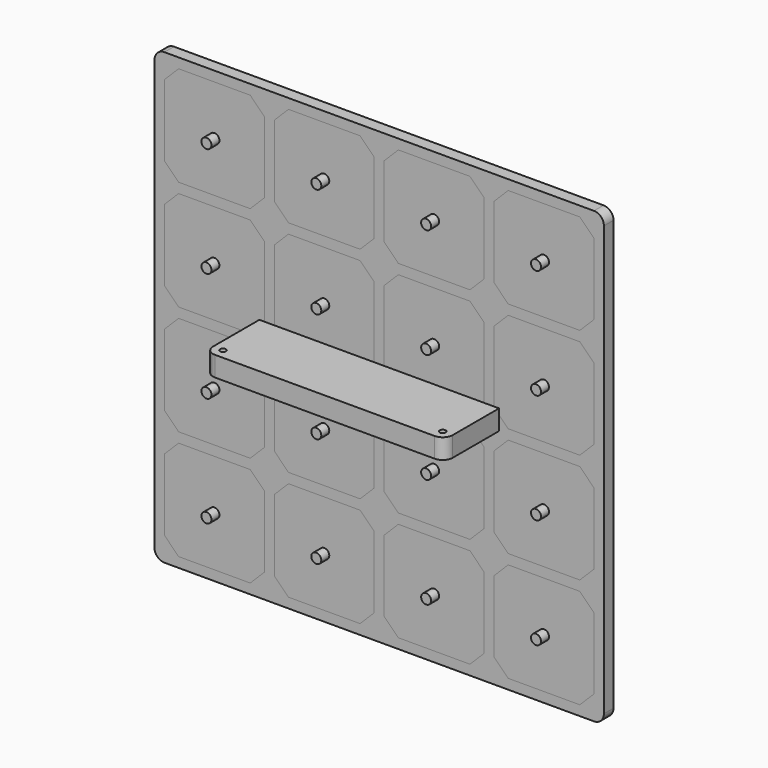
from build123d import *

# Parameters (mm, degrees)
F0_R          = 2.5
F1_DEPTH      = 6
F0_W          = 225
F0_H          = 225
F2_DEPTH      = 6
F3_R          = 5
F4_D          = 5
F4_2_D        = 5
F4_3_D        = 5
F4_4_D        = 5
F4_5_D        = 5
F4_6_D        = 5
F4_7_D        = 5
F4_8_D        = 5
F4_9_D        = 5
F4_10_D       = 5
F4_11_D       = 5
F4_12_D       = 5
F4_13_D       = 5
F4_14_D       = 5
F4_15_D       = 5
F5_R          = 2.5
F6_DEPTH      = 25
F6_DEPTH_BACK = 5
F8_DEPTH      = 10
F9_D          = 3
F10_T         = -3


with BuildPart() as f1:
    # F0 (on Front) → F1 (new body)
    with BuildSketch(Plane.XZ):
        Polygon((-107.5, 100.4289321881), (-107.5, 82.5), (-107.5, 64.5710678119), (-100.4289321881, 57.5), (-82.5, 57.5), (-64.5710678119, 57.5), (-57.5, 64.5710678119), (-57.5, 82.5), (-57.5, 100.4289321881), (-64.5710678119, 107.5), (-82.5, 107.5), (-100.4289321881, 107.5), align=None)
        with Locations((-82.5, 82.5)):
            Circle(F0_R, mode=Mode.SUBTRACT)
    extrude(amount=F1_DEPTH)


with BuildPart() as f1b:
    # F0 (on Front) → F1, piece 2 (new body)
    with BuildSketch(Plane.XZ):
        Polygon((-45.4289321881, 107.5), (-52.5, 100.4289321881), (-52.5, 82.5), (-52.5, 64.5710678119), (-45.4289321881, 57.5), (-27.5, 57.5), (-9.5710678119, 57.5), (-2.5, 64.5710678119), (-2.5, 82.5), (-2.5, 100.4289321881), (-9.5710678119, 107.5), (-27.5, 107.5), align=None)
    extrude(amount=F1_DEPTH)

    # F4 (through all)
    with Locations(Plane(origin=(0, 0, 0), x_dir=(1, 0, 0), z_dir=(0, 1, 0))):
        with Locations((-82.5, -82.5), (-27.5, -82.5), (27.5, -82.5), (82.5, -82.5), (-82.5, -27.5), (-27.5, -27.5), (27.5, -27.5), (82.5, -27.5), (-82.5, 27.5), (-27.5, 27.5), (27.5, 27.5), (82.5, 27.5), (-82.5, 82.5), (-27.5, 82.5), (27.5, 82.5), (82.5, 82.5)):
            Hole(F4_D / 2)


with BuildPart() as f1c:
    # F0 (on Front) → F1, piece 3 (new body)
    with BuildSketch(Plane.XZ):
        Polygon((9.5710678119, 107.5), (2.5, 100.4289321881), (2.5, 82.5), (2.5, 64.5710678119), (9.5710678119, 57.5), (27.5, 57.5), (45.4289321881, 57.5), (52.5, 64.5710678119), (52.5, 82.5), (52.5, 100.4289321881), (45.4289321881, 107.5), (27.5, 107.5), align=None)
    extrude(amount=F1_DEPTH)

    # F4#2 (through all)
    with Locations(Plane(origin=(0, 0, 0), x_dir=(1, 0, 0), z_dir=(0, 1, 0))):
        with Locations((-82.5, -82.5), (-27.5, -82.5), (27.5, -82.5), (82.5, -82.5), (-82.5, -27.5), (-27.5, -27.5), (27.5, -27.5), (82.5, -27.5), (-82.5, 27.5), (-27.5, 27.5), (27.5, 27.5), (82.5, 27.5), (-82.5, 82.5), (-27.5, 82.5), (27.5, 82.5), (82.5, 82.5)):
            Hole(F4_2_D / 2)


with BuildPart() as f1d:
    # F0 (on Front) → F1, piece 4 (new body)
    with BuildSketch(Plane.XZ):
        Polygon((64.5710678119, 107.5), (57.5, 100.4289321881), (57.5, 82.5), (57.5, 64.5710678119), (64.5710678119, 57.5), (82.5, 57.5), (100.4289321881, 57.5), (107.5, 64.5710678119), (107.5, 82.5), (107.5, 100.4289321881), (100.4289321881, 107.5), (82.5, 107.5), align=None)
    extrude(amount=F1_DEPTH)

    # F4#3 (through all)
    with Locations(Plane(origin=(0, 0, 0), x_dir=(1, 0, 0), z_dir=(0, 1, 0))):
        with Locations((-82.5, -82.5), (-27.5, -82.5), (27.5, -82.5), (82.5, -82.5), (-82.5, -27.5), (-27.5, -27.5), (27.5, -27.5), (82.5, -27.5), (-82.5, 27.5), (-27.5, 27.5), (27.5, 27.5), (82.5, 27.5), (-82.5, 82.5), (-27.5, 82.5), (27.5, 82.5), (82.5, 82.5)):
            Hole(F4_3_D / 2)


with BuildPart() as f1e:
    # F0 (on Front) → F1, piece 5 (new body)
    with BuildSketch(Plane.XZ):
        Polygon((64.5710678119, 52.5), (57.5, 45.4289321881), (57.5, 27.5), (57.5, 9.5710678119), (64.5710678119, 2.5), (82.5, 2.5), (100.4289321881, 2.5), (107.5, 9.5710678119), (107.5, 27.5), (107.5, 45.4289321881), (100.4289321881, 52.5), (82.5, 52.5), align=None)
    extrude(amount=F1_DEPTH)

    # F4#4 (through all)
    with Locations(Plane(origin=(0, 0, 0), x_dir=(1, 0, 0), z_dir=(0, 1, 0))):
        with Locations((-82.5, -82.5), (-27.5, -82.5), (27.5, -82.5), (82.5, -82.5), (-82.5, -27.5), (-27.5, -27.5), (27.5, -27.5), (82.5, -27.5), (-82.5, 27.5), (-27.5, 27.5), (27.5, 27.5), (82.5, 27.5), (-82.5, 82.5), (-27.5, 82.5), (27.5, 82.5), (82.5, 82.5)):
            Hole(F4_4_D / 2)


with BuildPart() as f1f:
    # F0 (on Front) → F1, piece 6 (new body)
    with BuildSketch(Plane.XZ):
        Polygon((9.5710678119, 52.5), (2.5, 45.4289321881), (2.5, 27.5), (2.5, 9.5710678119), (9.5710678119, 2.5), (27.5, 2.5), (45.4289321881, 2.5), (52.5, 9.5710678119), (52.5, 27.5), (52.5, 45.4289321881), (45.4289321881, 52.5), (27.5, 52.5), align=None)
    extrude(amount=F1_DEPTH)

    # F4#5 (through all)
    with Locations(Plane(origin=(0, 0, 0), x_dir=(1, 0, 0), z_dir=(0, 1, 0))):
        with Locations((-82.5, -82.5), (-27.5, -82.5), (27.5, -82.5), (82.5, -82.5), (-82.5, -27.5), (-27.5, -27.5), (27.5, -27.5), (82.5, -27.5), (-82.5, 27.5), (-27.5, 27.5), (27.5, 27.5), (82.5, 27.5), (-82.5, 82.5), (-27.5, 82.5), (27.5, 82.5), (82.5, 82.5)):
            Hole(F4_5_D / 2)


with BuildPart() as f1g:
    # F0 (on Front) → F1, piece 7 (new body)
    with BuildSketch(Plane.XZ):
        Polygon((-45.4289321881, 52.5), (-52.5, 45.4289321881), (-52.5, 27.5), (-52.5, 9.5710678119), (-45.4289321881, 2.5), (-27.5, 2.5), (-9.5710678119, 2.5), (-2.5, 9.5710678119), (-2.5, 27.5), (-2.5, 45.4289321881), (-9.5710678119, 52.5), (-27.5, 52.5), align=None)
    extrude(amount=F1_DEPTH)

    # F4#6 (through all)
    with Locations(Plane(origin=(0, 0, 0), x_dir=(1, 0, 0), z_dir=(0, 1, 0))):
        with Locations((-82.5, -82.5), (-27.5, -82.5), (27.5, -82.5), (82.5, -82.5), (-82.5, -27.5), (-27.5, -27.5), (27.5, -27.5), (82.5, -27.5), (-82.5, 27.5), (-27.5, 27.5), (27.5, 27.5), (82.5, 27.5), (-82.5, 82.5), (-27.5, 82.5), (27.5, 82.5), (82.5, 82.5)):
            Hole(F4_6_D / 2)


with BuildPart() as f1h:
    # F0 (on Front) → F1, piece 8 (new body)
    with BuildSketch(Plane.XZ):
        Polygon((-100.4289321881, 52.5), (-107.5, 45.4289321881), (-107.5, 27.5), (-107.5, 9.5710678119), (-100.4289321881, 2.5), (-82.5, 2.5), (-64.5710678119, 2.5), (-57.5, 9.5710678119), (-57.5, 27.5), (-57.5, 45.4289321881), (-64.5710678119, 52.5), (-82.5, 52.5), align=None)
    extrude(amount=F1_DEPTH)

    # F4#7 (through all)
    with Locations(Plane(origin=(0, 0, 0), x_dir=(1, 0, 0), z_dir=(0, 1, 0))):
        with Locations((-82.5, -82.5), (-27.5, -82.5), (27.5, -82.5), (82.5, -82.5), (-82.5, -27.5), (-27.5, -27.5), (27.5, -27.5), (82.5, -27.5), (-82.5, 27.5), (-27.5, 27.5), (27.5, 27.5), (82.5, 27.5), (-82.5, 82.5), (-27.5, 82.5), (27.5, 82.5), (82.5, 82.5)):
            Hole(F4_7_D / 2)


with BuildPart() as f1i:
    # F0 (on Front) → F1, piece 9 (new body)
    with BuildSketch(Plane.XZ):
        Polygon((-100.4289321881, -2.5), (-107.5, -9.5710678119), (-107.5, -27.5), (-107.5, -45.4289321881), (-100.4289321881, -52.5), (-82.5, -52.5), (-64.5710678119, -52.5), (-57.5, -45.4289321881), (-57.5, -27.5), (-57.5, -9.5710678119), (-64.5710678119, -2.5), (-82.5, -2.5), align=None)
    extrude(amount=F1_DEPTH)

    # F4#8 (through all)
    with Locations(Plane(origin=(0, 0, 0), x_dir=(1, 0, 0), z_dir=(0, 1, 0))):
        with Locations((-82.5, -82.5), (-27.5, -82.5), (27.5, -82.5), (82.5, -82.5), (-82.5, -27.5), (-27.5, -27.5), (27.5, -27.5), (82.5, -27.5), (-82.5, 27.5), (-27.5, 27.5), (27.5, 27.5), (82.5, 27.5), (-82.5, 82.5), (-27.5, 82.5), (27.5, 82.5), (82.5, 82.5)):
            Hole(F4_8_D / 2)


with BuildPart() as f1j:
    # F0 (on Front) → F1, piece 10 (new body)
    with BuildSketch(Plane.XZ):
        Polygon((-45.4289321881, -2.5), (-52.5, -9.5710678119), (-52.5, -27.5), (-52.5, -45.4289321881), (-45.4289321881, -52.5), (-27.5, -52.5), (-9.5710678119, -52.5), (-2.5, -45.4289321881), (-2.5, -27.5), (-2.5, -9.5710678119), (-9.5710678119, -2.5), (-27.5, -2.5), align=None)
    extrude(amount=F1_DEPTH)

    # F4#9 (through all)
    with Locations(Plane(origin=(0, 0, 0), x_dir=(1, 0, 0), z_dir=(0, 1, 0))):
        with Locations((-82.5, -82.5), (-27.5, -82.5), (27.5, -82.5), (82.5, -82.5), (-82.5, -27.5), (-27.5, -27.5), (27.5, -27.5), (82.5, -27.5), (-82.5, 27.5), (-27.5, 27.5), (27.5, 27.5), (82.5, 27.5), (-82.5, 82.5), (-27.5, 82.5), (27.5, 82.5), (82.5, 82.5)):
            Hole(F4_9_D / 2)


with BuildPart() as f1k:
    # F0 (on Front) → F1, piece 11 (new body)
    with BuildSketch(Plane.XZ):
        Polygon((9.5710678119, -2.5), (2.5, -9.5710678119), (2.5, -27.5), (2.5, -45.4289321881), (9.5710678119, -52.5), (27.5, -52.5), (45.4289321881, -52.5), (52.5, -45.4289321881), (52.5, -27.5), (52.5, -9.5710678119), (45.4289321881, -2.5), (27.5, -2.5), align=None)
    extrude(amount=F1_DEPTH)

    # F4#10 (through all)
    with Locations(Plane(origin=(0, 0, 0), x_dir=(1, 0, 0), z_dir=(0, 1, 0))):
        with Locations((-82.5, -82.5), (-27.5, -82.5), (27.5, -82.5), (82.5, -82.5), (-82.5, -27.5), (-27.5, -27.5), (27.5, -27.5), (82.5, -27.5), (-82.5, 27.5), (-27.5, 27.5), (27.5, 27.5), (82.5, 27.5), (-82.5, 82.5), (-27.5, 82.5), (27.5, 82.5), (82.5, 82.5)):
            Hole(F4_10_D / 2)


with BuildPart() as f1l:
    # F0 (on Front) → F1, piece 12 (new body)
    with BuildSketch(Plane.XZ):
        Polygon((64.5710678119, -2.5), (57.5, -9.5710678119), (57.5, -27.5), (57.5, -45.4289321881), (64.5710678119, -52.5), (82.5, -52.5), (100.4289321881, -52.5), (107.5, -45.4289321881), (107.5, -27.5), (107.5, -9.5710678119), (100.4289321881, -2.5), (82.5, -2.5), align=None)
    extrude(amount=F1_DEPTH)

    # F4#11 (through all)
    with Locations(Plane(origin=(0, 0, 0), x_dir=(1, 0, 0), z_dir=(0, 1, 0))):
        with Locations((-82.5, -82.5), (-27.5, -82.5), (27.5, -82.5), (82.5, -82.5), (-82.5, -27.5), (-27.5, -27.5), (27.5, -27.5), (82.5, -27.5), (-82.5, 27.5), (-27.5, 27.5), (27.5, 27.5), (82.5, 27.5), (-82.5, 82.5), (-27.5, 82.5), (27.5, 82.5), (82.5, 82.5)):
            Hole(F4_11_D / 2)


with BuildPart() as f1m:
    # F0 (on Front) → F1, piece 13 (new body)
    with BuildSketch(Plane.XZ):
        Polygon((64.5710678119, -57.5), (57.5, -64.5710678119), (57.5, -82.5), (57.5, -100.4289321881), (64.5710678119, -107.5), (82.5, -107.5), (100.4289321881, -107.5), (107.5, -100.4289321881), (107.5, -82.5), (107.5, -64.5710678119), (100.4289321881, -57.5), (82.5, -57.5), align=None)
    extrude(amount=F1_DEPTH)

    # F4#12 (through all)
    with Locations(Plane(origin=(0, 0, 0), x_dir=(1, 0, 0), z_dir=(0, 1, 0))):
        with Locations((-82.5, -82.5), (-27.5, -82.5), (27.5, -82.5), (82.5, -82.5), (-82.5, -27.5), (-27.5, -27.5), (27.5, -27.5), (82.5, -27.5), (-82.5, 27.5), (-27.5, 27.5), (27.5, 27.5), (82.5, 27.5), (-82.5, 82.5), (-27.5, 82.5), (27.5, 82.5), (82.5, 82.5)):
            Hole(F4_12_D / 2)


with BuildPart() as f1n:
    # F0 (on Front) → F1, piece 14 (new body)
    with BuildSketch(Plane.XZ):
        Polygon((9.5710678119, -57.5), (2.5, -64.5710678119), (2.5, -82.5), (2.5, -100.4289321881), (9.5710678119, -107.5), (27.5, -107.5), (45.4289321881, -107.5), (52.5, -100.4289321881), (52.5, -82.5), (52.5, -64.5710678119), (45.4289321881, -57.5), (27.5, -57.5), align=None)
    extrude(amount=F1_DEPTH)

    # F4#13 (through all)
    with Locations(Plane(origin=(0, 0, 0), x_dir=(1, 0, 0), z_dir=(0, 1, 0))):
        with Locations((-82.5, -82.5), (-27.5, -82.5), (27.5, -82.5), (82.5, -82.5), (-82.5, -27.5), (-27.5, -27.5), (27.5, -27.5), (82.5, -27.5), (-82.5, 27.5), (-27.5, 27.5), (27.5, 27.5), (82.5, 27.5), (-82.5, 82.5), (-27.5, 82.5), (27.5, 82.5), (82.5, 82.5)):
            Hole(F4_13_D / 2)


with BuildPart() as f1o:
    # F0 (on Front) → F1, piece 15 (new body)
    with BuildSketch(Plane.XZ):
        Polygon((-45.4289321881, -57.5), (-52.5, -64.5710678119), (-52.5, -82.5), (-52.5, -100.4289321881), (-45.4289321881, -107.5), (-27.5, -107.5), (-9.5710678119, -107.5), (-2.5, -100.4289321881), (-2.5, -82.5), (-2.5, -64.5710678119), (-9.5710678119, -57.5), (-27.5, -57.5), align=None)
    extrude(amount=F1_DEPTH)

    # F4#14 (through all)
    with Locations(Plane(origin=(0, 0, 0), x_dir=(1, 0, 0), z_dir=(0, 1, 0))):
        with Locations((-82.5, -82.5), (-27.5, -82.5), (27.5, -82.5), (82.5, -82.5), (-82.5, -27.5), (-27.5, -27.5), (27.5, -27.5), (82.5, -27.5), (-82.5, 27.5), (-27.5, 27.5), (27.5, 27.5), (82.5, 27.5), (-82.5, 82.5), (-27.5, 82.5), (27.5, 82.5), (82.5, 82.5)):
            Hole(F4_14_D / 2)


with BuildPart() as f1p:
    # F0 (on Front) → F1, piece 16 (new body)
    with BuildSketch(Plane.XZ):
        Polygon((-100.4289321881, -57.5), (-107.5, -64.5710678119), (-107.5, -82.5), (-107.5, -100.4289321881), (-100.4289321881, -107.5), (-82.5, -107.5), (-64.5710678119, -107.5), (-57.5, -100.4289321881), (-57.5, -82.5), (-57.5, -64.5710678119), (-64.5710678119, -57.5), (-82.5, -57.5), align=None)
    extrude(amount=F1_DEPTH)

    # F4#15 (through all)
    with Locations(Plane(origin=(0, 0, 0), x_dir=(1, 0, 0), z_dir=(0, 1, 0))):
        with Locations((-82.5, -82.5), (-27.5, -82.5), (27.5, -82.5), (82.5, -82.5), (-82.5, -27.5), (-27.5, -27.5), (27.5, -27.5), (82.5, -27.5), (-82.5, 27.5), (-27.5, 27.5), (27.5, 27.5), (82.5, 27.5), (-82.5, 82.5), (-27.5, 82.5), (27.5, 82.5), (82.5, 82.5)):
            Hole(F4_15_D / 2)


with BuildPart() as f2:
    # F0 (on Front) → F2 (new body)
    with BuildSketch(Plane.XZ):
        Rectangle(F0_W, F0_H)
        Polygon((-107.5, -82.5), (-107.5, -64.5710678119), (-100.4289321881, -57.5), (-82.5, -57.5), (-64.5710678119, -57.5), (-57.5, -64.5710678119), (-57.5, -82.5), (-57.5, -100.4289321881), (-64.5710678119, -107.5), (-82.5, -107.5), (-100.4289321881, -107.5), (-107.5, -100.4289321881), align=None, mode=Mode.SUBTRACT)
        Polygon((-52.5, -82.5), (-52.5, -64.5710678119), (-45.4289321881, -57.5), (-27.5, -57.5), (-9.5710678119, -57.5), (-2.5, -64.5710678119), (-2.5, -82.5), (-2.5, -100.4289321881), (-9.5710678119, -107.5), (-27.5, -107.5), (-45.4289321881, -107.5), (-52.5, -100.4289321881), align=None, mode=Mode.SUBTRACT)
        Polygon((-107.5, -27.5), (-107.5, -9.5710678119), (-100.4289321881, -2.5), (-82.5, -2.5), (-64.5710678119, -2.5), (-57.5, -9.5710678119), (-57.5, -27.5), (-57.5, -45.4289321881), (-64.5710678119, -52.5), (-82.5, -52.5), (-100.4289321881, -52.5), (-107.5, -45.4289321881), align=None, mode=Mode.SUBTRACT)
        Polygon((-52.5, -27.5), (-52.5, -9.5710678119), (-45.4289321881, -2.5), (-27.5, -2.5), (-9.5710678119, -2.5), (-2.5, -9.5710678119), (-2.5, -27.5), (-2.5, -45.4289321881), (-9.5710678119, -52.5), (-27.5, -52.5), (-45.4289321881, -52.5), (-52.5, -45.4289321881), align=None, mode=Mode.SUBTRACT)
        Polygon((2.5, -82.5), (2.5, -64.5710678119), (9.5710678119, -57.5), (27.5, -57.5), (45.4289321881, -57.5), (52.5, -64.5710678119), (52.5, -82.5), (52.5, -100.4289321881), (45.4289321881, -107.5), (27.5, -107.5), (9.5710678119, -107.5), (2.5, -100.4289321881), align=None, mode=Mode.SUBTRACT)
        Polygon((57.5, -82.5), (57.5, -64.5710678119), (64.5710678119, -57.5), (82.5, -57.5), (100.4289321881, -57.5), (107.5, -64.5710678119), (107.5, -82.5), (107.5, -100.4289321881), (100.4289321881, -107.5), (82.5, -107.5), (64.5710678119, -107.5), (57.5, -100.4289321881), align=None, mode=Mode.SUBTRACT)
        Polygon((2.5, -27.5), (2.5, -9.5710678119), (9.5710678119, -2.5), (27.5, -2.5), (45.4289321881, -2.5), (52.5, -9.5710678119), (52.5, -27.5), (52.5, -45.4289321881), (45.4289321881, -52.5), (27.5, -52.5), (9.5710678119, -52.5), (2.5, -45.4289321881), align=None, mode=Mode.SUBTRACT)
        Polygon((57.5, -27.5), (57.5, -9.5710678119), (64.5710678119, -2.5), (82.5, -2.5), (100.4289321881, -2.5), (107.5, -9.5710678119), (107.5, -27.5), (107.5, -45.4289321881), (100.4289321881, -52.5), (82.5, -52.5), (64.5710678119, -52.5), (57.5, -45.4289321881), align=None, mode=Mode.SUBTRACT)
        Polygon((-107.5, 27.5), (-107.5, 45.4289321881), (-100.4289321881, 52.5), (-82.5, 52.5), (-64.5710678119, 52.5), (-57.5, 45.4289321881), (-57.5, 27.5), (-57.5, 9.5710678119), (-64.5710678119, 2.5), (-82.5, 2.5), (-100.4289321881, 2.5), (-107.5, 9.5710678119), align=None, mode=Mode.SUBTRACT)
        Polygon((-52.5, 27.5), (-52.5, 45.4289321881), (-45.4289321881, 52.5), (-27.5, 52.5), (-9.5710678119, 52.5), (-2.5, 45.4289321881), (-2.5, 27.5), (-2.5, 9.5710678119), (-9.5710678119, 2.5), (-27.5, 2.5), (-45.4289321881, 2.5), (-52.5, 9.5710678119), align=None, mode=Mode.SUBTRACT)
        Polygon((-107.5, 64.5710678119), (-107.5, 82.5), (-107.5, 100.4289321881), (-100.4289321881, 107.5), (-82.5, 107.5), (-64.5710678119, 107.5), (-57.5, 100.4289321881), (-57.5, 82.5), (-57.5, 64.5710678119), (-64.5710678119, 57.5), (-82.5, 57.5), (-100.4289321881, 57.5), align=None, mode=Mode.SUBTRACT)
        Polygon((-52.5, 82.5), (-52.5, 100.4289321881), (-45.4289321881, 107.5), (-27.5, 107.5), (-9.5710678119, 107.5), (-2.5, 100.4289321881), (-2.5, 82.5), (-2.5, 64.5710678119), (-9.5710678119, 57.5), (-27.5, 57.5), (-45.4289321881, 57.5), (-52.5, 64.5710678119), align=None, mode=Mode.SUBTRACT)
        Polygon((2.5, 27.5), (2.5, 45.4289321881), (9.5710678119, 52.5), (27.5, 52.5), (45.4289321881, 52.5), (52.5, 45.4289321881), (52.5, 27.5), (52.5, 9.5710678119), (45.4289321881, 2.5), (27.5, 2.5), (9.5710678119, 2.5), (2.5, 9.5710678119), align=None, mode=Mode.SUBTRACT)
        Polygon((57.5, 27.5), (57.5, 45.4289321881), (64.5710678119, 52.5), (82.5, 52.5), (100.4289321881, 52.5), (107.5, 45.4289321881), (107.5, 27.5), (107.5, 9.5710678119), (100.4289321881, 2.5), (82.5, 2.5), (64.5710678119, 2.5), (57.5, 9.5710678119), align=None, mode=Mode.SUBTRACT)
        Polygon((2.5, 82.5), (2.5, 100.4289321881), (9.5710678119, 107.5), (27.5, 107.5), (45.4289321881, 107.5), (52.5, 100.4289321881), (52.5, 82.5), (52.5, 64.5710678119), (45.4289321881, 57.5), (27.5, 57.5), (9.5710678119, 57.5), (2.5, 64.5710678119), align=None, mode=Mode.SUBTRACT)
        Polygon((57.5, 82.5), (57.5, 100.4289321881), (64.5710678119, 107.5), (82.5, 107.5), (100.4289321881, 107.5), (107.5, 100.4289321881), (107.5, 82.5), (107.5, 64.5710678119), (100.4289321881, 57.5), (82.5, 57.5), (64.5710678119, 57.5), (57.5, 64.5710678119), align=None, mode=Mode.SUBTRACT)
    extrude(amount=F2_DEPTH)

    # F3
    f3_edges = [f2.edges().sort_by_distance(p)[0] for p in [
        (-112.5, -3, 112.5),
        (112.5, -3, 112.5),
        (112.5, -3, -112.5),
        (-112.5, -3, -112.5),
    ]]
    fillet(f3_edges, radius=F3_R)


with BuildPart() as f6:
    # F5 (on face) → F6 (new body, two sides)
    with BuildSketch(Plane.XZ.offset(6)) as f6_sk:
        with Locations((-82.5, 82.5)):
            Circle(F5_R)
    extrude(amount=-F6_DEPTH)
    extrude(f6_sk.sketch, amount=F6_DEPTH_BACK)


with BuildPart() as f6b:
    # F5 (on face) → F6, piece 2 (new body, two sides)
    with BuildSketch(Plane.XZ.offset(6)) as f6_2_sk:
        with Locations((-82.5, 27.5)):
            Circle(F5_R)
    extrude(amount=-F6_DEPTH)
    extrude(f6_2_sk.sketch, amount=F6_DEPTH_BACK)


with BuildPart() as f6c:
    # F5 (on face) → F6, piece 3 (new body, two sides)
    with BuildSketch(Plane.XZ.offset(6)) as f6_3_sk:
        with Locations((-82.5, -27.5)):
            Circle(F5_R)
    extrude(amount=-F6_DEPTH)
    extrude(f6_3_sk.sketch, amount=F6_DEPTH_BACK)


with BuildPart() as f6d:
    # F5 (on face) → F6, piece 4 (new body, two sides)
    with BuildSketch(Plane.XZ.offset(6)) as f6_4_sk:
        with Locations((-82.5, -82.5)):
            Circle(F5_R)
    extrude(amount=-F6_DEPTH)
    extrude(f6_4_sk.sketch, amount=F6_DEPTH_BACK)


with BuildPart() as f6e:
    # F5 (on face) → F6, piece 5 (new body, two sides)
    with BuildSketch(Plane.XZ.offset(6)) as f6_5_sk:
        with Locations((-27.5, 82.5)):
            Circle(F5_R)
    extrude(amount=-F6_DEPTH)
    extrude(f6_5_sk.sketch, amount=F6_DEPTH_BACK)


with BuildPart() as f6f:
    # F5 (on face) → F6, piece 6 (new body, two sides)
    with BuildSketch(Plane.XZ.offset(6)) as f6_6_sk:
        with Locations((-27.5, 27.5)):
            Circle(F5_R)
    extrude(amount=-F6_DEPTH)
    extrude(f6_6_sk.sketch, amount=F6_DEPTH_BACK)


with BuildPart() as f6g:
    # F5 (on face) → F6, piece 7 (new body, two sides)
    with BuildSketch(Plane.XZ.offset(6)) as f6_7_sk:
        with Locations((-27.5, -27.5)):
            Circle(F5_R)
    extrude(amount=-F6_DEPTH)
    extrude(f6_7_sk.sketch, amount=F6_DEPTH_BACK)


with BuildPart() as f6h:
    # F5 (on face) → F6, piece 8 (new body, two sides)
    with BuildSketch(Plane.XZ.offset(6)) as f6_8_sk:
        with Locations((-27.5, -82.5)):
            Circle(F5_R)
    extrude(amount=-F6_DEPTH)
    extrude(f6_8_sk.sketch, amount=F6_DEPTH_BACK)


with BuildPart() as f6i:
    # F5 (on face) → F6, piece 9 (new body, two sides)
    with BuildSketch(Plane.XZ.offset(6)) as f6_9_sk:
        with Locations((27.5, 82.5)):
            Circle(F5_R)
    extrude(amount=-F6_DEPTH)
    extrude(f6_9_sk.sketch, amount=F6_DEPTH_BACK)


with BuildPart() as f6j:
    # F5 (on face) → F6, piece 10 (new body, two sides)
    with BuildSketch(Plane.XZ.offset(6)) as f6_10_sk:
        with Locations((27.5, 27.5)):
            Circle(F5_R)
    extrude(amount=-F6_DEPTH)
    extrude(f6_10_sk.sketch, amount=F6_DEPTH_BACK)


with BuildPart() as f6k:
    # F5 (on face) → F6, piece 11 (new body, two sides)
    with BuildSketch(Plane.XZ.offset(6)) as f6_11_sk:
        with Locations((27.5, -27.5)):
            Circle(F5_R)
    extrude(amount=-F6_DEPTH)
    extrude(f6_11_sk.sketch, amount=F6_DEPTH_BACK)


with BuildPart() as f6l:
    # F5 (on face) → F6, piece 12 (new body, two sides)
    with BuildSketch(Plane.XZ.offset(6)) as f6_12_sk:
        with Locations((27.5, -82.5)):
            Circle(F5_R)
    extrude(amount=-F6_DEPTH)
    extrude(f6_12_sk.sketch, amount=F6_DEPTH_BACK)


with BuildPart() as f6m:
    # F5 (on face) → F6, piece 13 (new body, two sides)
    with BuildSketch(Plane.XZ.offset(6)) as f6_13_sk:
        with Locations((82.5, 82.5)):
            Circle(F5_R)
    extrude(amount=-F6_DEPTH)
    extrude(f6_13_sk.sketch, amount=F6_DEPTH_BACK)


with BuildPart() as f6n:
    # F5 (on face) → F6, piece 14 (new body, two sides)
    with BuildSketch(Plane.XZ.offset(6)) as f6_14_sk:
        with Locations((82.5, 27.5)):
            Circle(F5_R)
    extrude(amount=-F6_DEPTH)
    extrude(f6_14_sk.sketch, amount=F6_DEPTH_BACK)


with BuildPart() as f6o:
    # F5 (on face) → F6, piece 15 (new body, two sides)
    with BuildSketch(Plane.XZ.offset(6)) as f6_15_sk:
        with Locations((82.5, -27.5)):
            Circle(F5_R)
    extrude(amount=-F6_DEPTH)
    extrude(f6_15_sk.sketch, amount=F6_DEPTH_BACK)


with BuildPart() as f6p:
    # F5 (on face) → F6, piece 16 (new body, two sides)
    with BuildSketch(Plane.XZ.offset(6)) as f6_16_sk:
        with Locations((82.5, -82.5)):
            Circle(F5_R)
    extrude(amount=-F6_DEPTH)
    extrude(f6_16_sk.sketch, amount=F6_DEPTH_BACK)


with BuildPart() as f8:
    # F7 (on Top) → F8 (new body)
    with BuildSketch(Plane.XY):
        with BuildLine():
            Line((55, 40), (-55, 40))
            ThreePointArc((-55, 40), (-58.5355339059, 38.5355339059), (-60, 35))
            Line((-60, 35), (-60, -35))
            ThreePointArc((-60, -35), (-58.5355339059, -38.5355339059), (-55, -40))
            Line((-55, -40), (55, -40))
            ThreePointArc((55, -40), (58.5355339059, -38.5355339059), (60, -35))
            Line((60, -35), (60, 35))
            ThreePointArc((60, 35), (58.5355339059, 38.5355339059), (55, 40))
        make_face()
    extrude(amount=F8_DEPTH)

    # F9 (through all)
    with Locations(Plane(origin=(0, 0, 0), x_dir=(1, 0, 0), z_dir=(0, 0, -1))):
        with Locations((-55, -35), (55, -35), (55, 35), (-55, 35)):
            Hole(F9_D / 2)

    # F10
    f10_openings = [f8.faces().sort_by_distance(p)[0] for p in [
        (0, 0, 0),
    ]]
    offset(amount=F10_T, openings=f10_openings)


solid = Compound([f1.part, f1b.part, f1c.part, f1d.part, f1e.part, f1f.part, f1g.part, f1h.part, f1i.part, f1j.part, f1k.part, f1l.part, f1m.part, f1n.part, f1o.part, f1p.part, f2.part, f6.part, f6b.part, f6c.part, f6d.part, f6e.part, f6f.part, f6g.part, f6h.part, f6i.part, f6j.part, f6k.part, f6l.part, f6m.part, f6n.part, f6o.part, f6p.part, f8.part])
